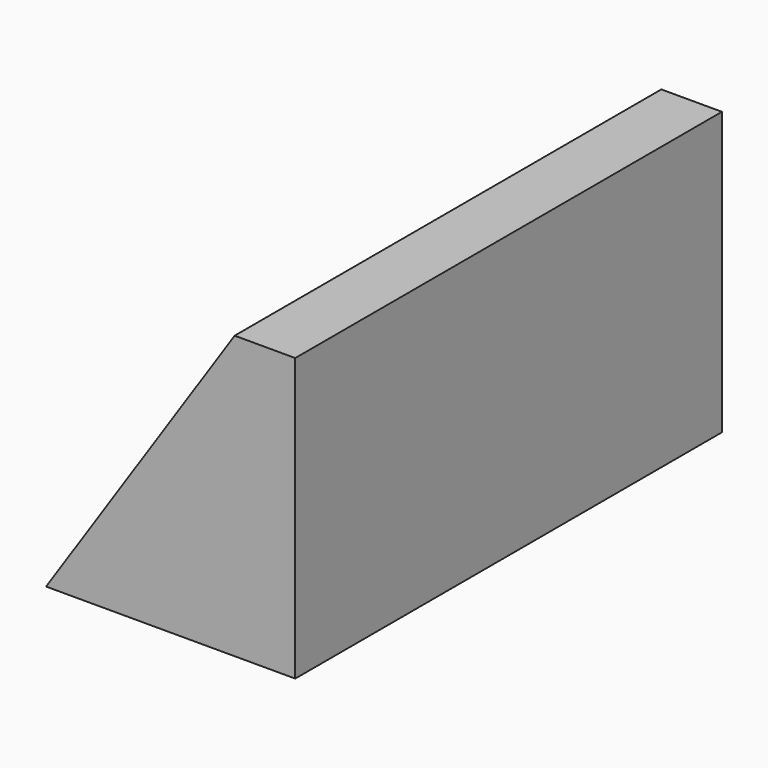
from build123d import *

# Parameters (mm, degrees)
F1_DEPTH = 55.88


# Not quite as in the source:
# - a feature names something its author has since deleted; it is built from what else it names


with BuildPart() as f1:
    # F0 (on Front) → F1 (new body)
    with BuildSketch(Plane.XZ):
        Polygon((-26.1060774862, 0), (0, 0), (0, 29.5670594135), (-6.35, 29.5670594135), align=None)
    extrude(amount=F1_DEPTH)


solid = f1.part
